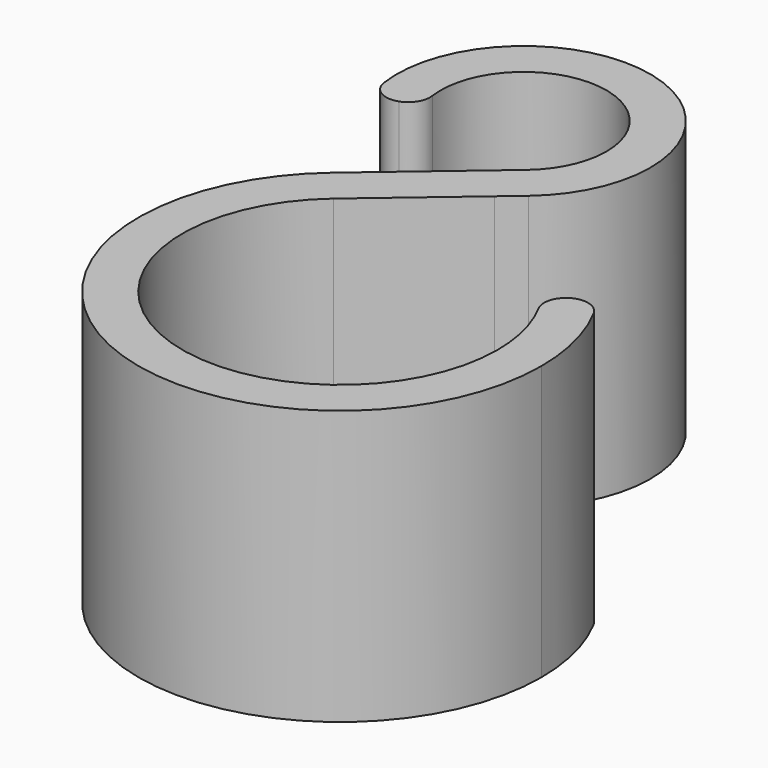
from build123d import *

# Parameters (mm, degrees)
F1_DEPTH = 20
F2_R     = 1.59999


# Not quite as in the source:
# - a fillet or chamfer is up to 0.001 mm smaller than in the source, because OpenCascade refuses the exact size


with BuildPart() as f1:
    # F0 (on Top) → F1 (new body)
    with BuildSketch(Plane.XY):
        with BuildLine():
            ThreePointArc((6.05, 0), (5.4927369002, -2.5362060928), (3.9236061669, -4.6051943115))
            Line((3.9236061669, -4.6051943115), (-1.4025425598, -9.1430506051))
            ThreePointArc((-1.4025425598, -9.1430506051), (-0.799716174, -9.2153651062), (-0.1934443699, -9.2479770369))
            ThreePointArc((-0.1934443699, -9.2479770369), (1.8772842283, -8.6355074503), (4.015398341, -8.3330112302))
            ThreePointArc((4.015398341, -8.3330112302), (5.0486509404, -7.7507176237), (5.9989019907, -7.0409995672))
            ThreePointArc((5.9989019907, -7.0409995672), (8.3979861697, -3.8776704725), (9.25, 0))
            ThreePointArc((9.25, 0), (-1.6062456434, 9.1094717154), (-8.6921567423, -3.1636863258))
            Line((-8.6921567423, -3.1636863258), (-5.6851403558, -2.0692218671))
            ThreePointArc((-5.6851403558, -2.0692218671), (-1.0505714749, 5.9580869057), (6.05, 0))
        make_face()
        with BuildLine():
            ThreePointArc((4.015398341, -8.3330112302), (1.9649742101, -9.0388813663), (-0.1934443699, -9.2479770369))
            ThreePointArc((-0.1934443699, -9.2479770369), (-2.4740598171, -10.3418630972), (-4.5333901906, -11.8105196067))
            ThreePointArc((-4.5333901906, -11.8105196067), (-1.1623519941, -36.3459888319), (19.7, -23))
            ThreePointArc((19.7, -23), (19.0087472673, -18.5452272785), (17, -14.5094169811))
            Line((17, -14.5094169811), (14.387755102, -16.3577071621))
            ThreePointArc((14.387755102, -16.3577071621), (15.9592240527, -19.5149737213), (16.5, -23))
            ThreePointArc((16.5, -23), (0.1791123856, -33.4407395624), (-2.4580943668, -14.2463248624))
            Line((-2.4580943668, -14.2463248624), (4.5116719892, -8.3081132677))
            ThreePointArc((4.5116719892, -8.3081132677), (4.2634299557, -8.3184651834), (4.015398341, -8.3330112302))
        make_face()
        with BuildLine():
            ThreePointArc((-0.1934443699, -9.2479770369), (-0.799716174, -9.2153651062), (-1.4025425598, -9.1430506051))
            Line((-1.4025425598, -9.1430506051), (-4.5333901906, -11.8105196067))
            ThreePointArc((-4.5333901906, -11.8105196067), (-2.4740598171, -10.3418630972), (-0.1934443699, -9.2479770369))
        make_face()
        with BuildLine():
            ThreePointArc((4.015398341, -8.3330112302), (1.8772842283, -8.6355074503), (-0.1934443699, -9.2479770369))
            ThreePointArc((-0.1934443699, -9.2479770369), (1.9649742101, -9.0388813663), (4.015398341, -8.3330112302))
        make_face()
        with BuildLine():
            ThreePointArc((5.9989019907, -7.0409995672), (5.0486509404, -7.7507176237), (4.015398341, -8.3330112302))
            ThreePointArc((4.015398341, -8.3330112302), (4.2634299557, -8.3184651834), (4.5116719892, -8.3081132677))
            Line((4.5116719892, -8.3081132677), (5.9989019907, -7.0409995672))
        make_face()
    extrude(amount=F1_DEPTH)

    # F2 (radius 1.6 in the source; OpenCascade refuses exactly that, so slightly less here)
    f2_edges = [f1.edges().sort_by_distance(p)[0] for p in [
        (17, -14.509417, 10),
        (14.387755, -16.357707, 10),
        (-8.692157, -3.163686, 10),
        (-5.68514, -2.069222, 10),
    ]]
    fillet(f2_edges, radius=F2_R)


solid = f1.part
